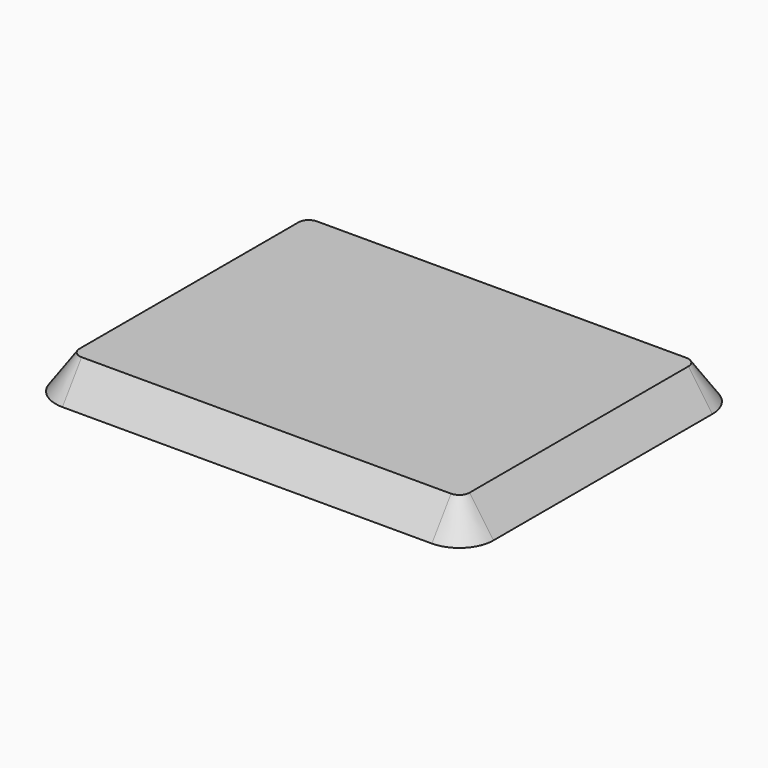
from build123d import *

# Parameters (mm, degrees)
F0_W     = 32
F0_H     = 25
F1_DEPTH = 2.5
F2_R     = 2.5
F3_SIZE2 = 2.49999
F3_SIZE  = 1.750509


# Not quite as in the source:
# - a fillet or chamfer is up to 0.001 mm smaller than in the source, because OpenCascade refuses the exact size


with BuildPart() as f1:
    # F0 (on Top) → F1 (new body)
    with BuildSketch(Plane.XY):
        Rectangle(F0_W, F0_H)
    extrude(amount=F1_DEPTH)

    # F2
    f2_edges = [f1.edges().sort_by_distance(p)[0] for p in [
        (-16, -12.5, 1.25),
        (16, -12.5, 1.25),
        (16, 12.5, 1.25),
        (-16, 12.5, 1.25),
    ]]
    fillet(f2_edges, radius=F2_R)

    # F3 (size 1.7505188455 and 2.5 in the source; OpenCascade refuses exactly that, so slightly less here)
    f3_edges = [f1.edges().sort_by_distance(p)[0] for p in [
        (0, -12.5, 2.5),
        (-16, 0, 2.5),
        (15.267767, -11.767767, 2.5),
        (16, 0, 2.5),
        (15.267767, 11.767767, 2.5),
        (0, 12.5, 2.5),
        (-15.267767, 11.767767, 2.5),
        (-15.267767, -11.767767, 2.5),
    ]]
    f3_side = f1.faces().sort_by_distance((0, 0, 2.5))[0]
    chamfer(f3_edges, length=F3_SIZE, length2=F3_SIZE2, reference=f3_side)


solid = f1.part
